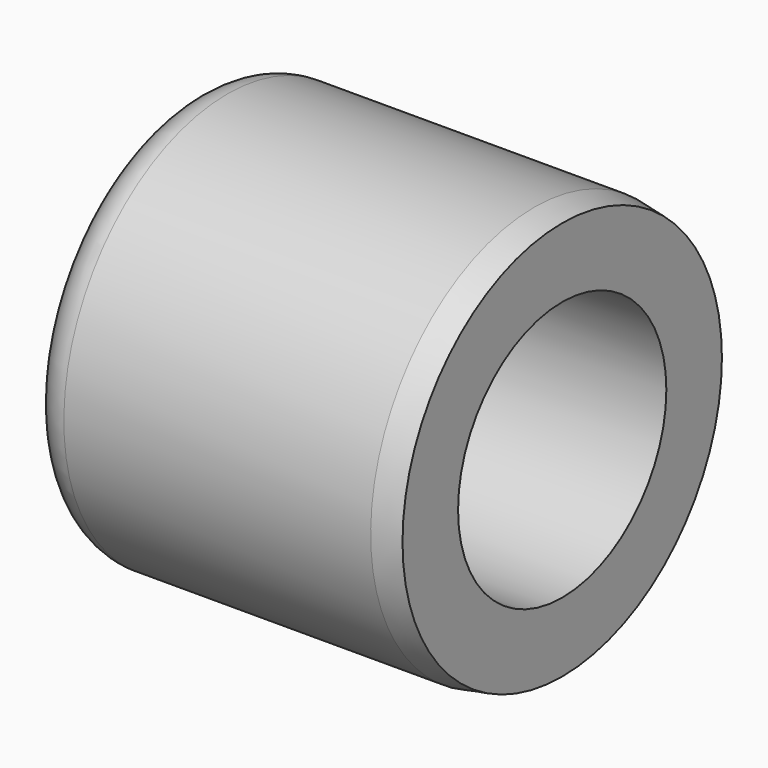
from build123d import *

# Parameters (mm, degrees)
F0_W = 20
F0_H = 4
F4_R = 1.99999


# Not quite as in the source:
# - a fillet or chamfer is up to 0.001 mm smaller than in the source, because OpenCascade refuses the exact size


with BuildPart() as f1:
    # F0 (on Front) → F1 (revolve)
    with BuildSketch(Plane.XZ):
        with Locations((10, 9)):
            Rectangle(F0_W, F0_H)
    revolve(axis=Axis((12.6487514935, 0, 0), (1, 0, 0)))

    # F2 (on Front) → F3 (revolve, cut)
    with BuildSketch(Plane.XZ):
        Polygon((24, 11.9697983939), (13, 11.9697983939), (24, 10.0302016061), align=None)
    revolve(axis=Axis((11.270377785, 0, 0), (1, 0, 0)), mode=Mode.SUBTRACT)

    # F4 (radius 2 in the source; OpenCascade refuses exactly that, so slightly less here)
    f4_edges = [f1.edges().sort_by_distance(p)[0] for p in [
        (0, 0, -11),
        (0, 0, -7),
    ]]
    fillet(f4_edges, radius=F4_R)


solid = f1.part
